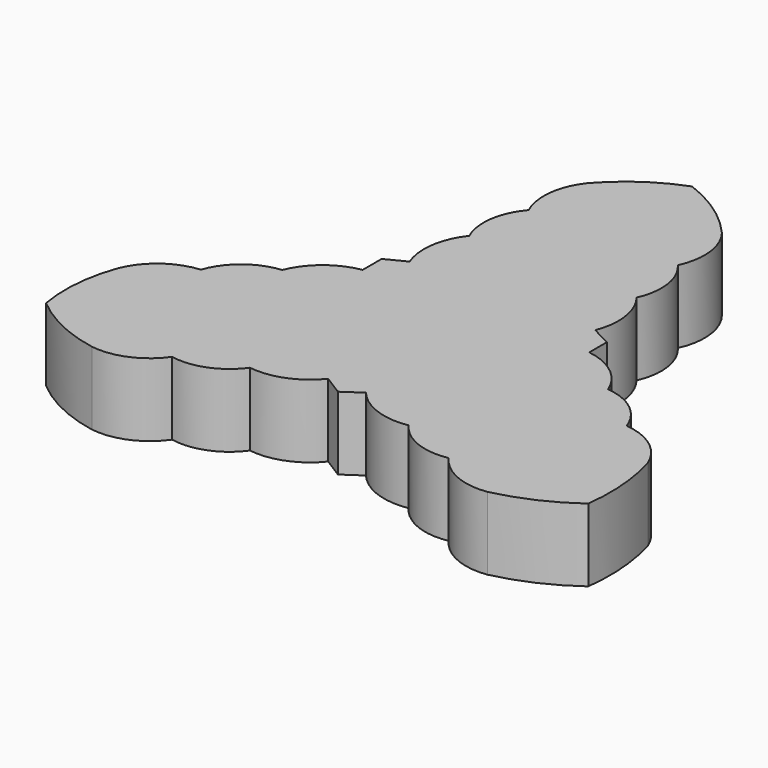
from build123d import *

# Parameters (mm, degrees)
F1_DEPTH = 7.9375


# Not quite as in the source:
# - a length typed as a fraction of an inch, garbled in the dataset ("3 / 203.2 mm" for 3/8 in), is restored


with BuildPart() as f1:
    # F0 (on Top) → F1 (new body)
    with BuildSketch(Plane.XY):
        with BuildLine():
            ThreePointArc((-0.0986067535, 34.0497419238), (-4.0682176485, 31.9659465467), (-7.4162920937, 28.9842672646))
            ThreePointArc((-7.4162920937, 28.9842672646), (-8.8119305122, 25.5953281623), (-8.2258973271, 21.977417171))
            ThreePointArc((-8.2258973271, 21.977417171), (-9.7181261566, 18.698842434), (-9.2097157612, 15.1327075437))
            ThreePointArc((-9.2097157612, 15.1327075437), (-10.6205392688, 11.8246856933), (-10.2093555033, 8.2519613206))
            Line((-10.2093555033, 8.2519613206), (-12.369341217, 7.1464567445))
            Line((-12.369341217, 7.1464567445), (-12.369341217, 4.6386048198))
            Line((-12.369341217, 4.6386048198), (-12.369341217, 4.5682978211))
            ThreePointArc((-12.369341217, 4.5682978211), (-15.5930977879, 3.1185654947), (-17.7027139134, 0.2823972963))
            ThreePointArc((-17.7027139134, 0.2823972963), (-21.0452825194, -1.0603738309), (-23.1384971151, -3.9919692741))
            ThreePointArc((-23.1384971151, -3.9919692741), (-26.5647165348, -5.2934051439), (-28.80180468, -8.19653302))
            ThreePointArc((-28.80180468, -8.19653302), (-29.7673344436, -12.5572908836), (-29.5614041388, -17.0189104974))
            ThreePointArc((-29.5614041388, -17.0189104974), (-25.7783661022, -19.4669407743), (-21.4921734029, -20.8571857766))
            ThreePointArc((-21.4921734029, -20.8571857766), (-17.8594468391, -20.3713745504), (-15.0192606046, -18.054899429))
            ThreePointArc((-15.0192606046, -18.054899429), (-11.4338171794, -17.7079201351), (-8.5996589687, -15.484556372))
            ThreePointArc((-8.5996589687, -15.484556372), (-5.0294162563, -15.0523544446), (-2.1409380715, -12.9098966718))
            Line((-2.1409380715, -12.9098966718), (0, -14.2561570176))
            Line((0, -14.2561570176), (1.9696742658, -12.9098966718))
            ThreePointArc((1.9696742658, -12.9098966718), (4.9392756736, -15.0084468105), (8.560301624, -15.3410370587))
            ThreePointArc((8.560301624, -15.3410370587), (11.3944598347, -17.5644008218), (14.9799032599, -17.9113801157))
            ThreePointArc((14.9799032599, -17.9113801157), (17.8200894944, -20.2278552371), (21.4528160582, -20.7136664634))
            ThreePointArc((21.4528160582, -20.7136664634), (25.6558468929, -19.2922500665), (29.4813849032, -17.0447733253))
            ThreePointArc((29.4813849032, -17.0447733253), (29.5836204245, -12.511977875), (28.7624473353, -8.0530137067))
            ThreePointArc((28.7624473353, -8.0530137067), (26.5253591901, -5.1498858306), (23.0991397704, -3.8484499608))
            ThreePointArc((23.0991397704, -3.8484499608), (21.0059251747, -0.9168545176), (17.6633565687, 0.4259166096))
            ThreePointArc((17.6633565687, 0.4259166096), (15.4847616458, 3.3168082822), (12.1560195839, 4.739132713))
            Line((12.1560195839, 4.739132713), (12.1560195839, 7.1464567445))
            Line((12.1560195839, 7.1464567445), (9.9960338703, 8.2519613206))
            ThreePointArc((9.9960338703, 8.2519613206), (10.4072176357, 11.8246856933), (8.9963941282, 15.1327075437))
            ThreePointArc((8.9963941282, 15.1327075437), (9.5048045235, 18.698842434), (8.012575694, 21.977417171))
            ThreePointArc((8.012575694, 21.977417171), (8.5986088792, 25.5953281623), (7.2029704606, 28.9842672646))
            ThreePointArc((7.2029704606, 28.9842672646), (3.8655773676, 31.9687453881), (-0.0986067535, 34.0497419238))
        make_face()
    extrude(amount=F1_DEPTH)


solid = f1.part
